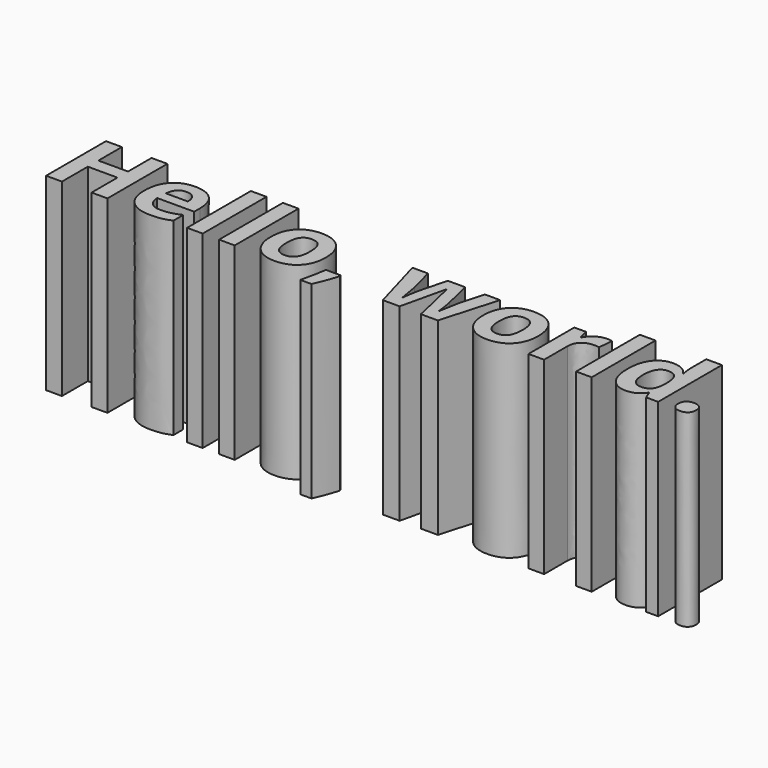
from build123d import *

# Parameters (mm, degrees)
F0_TEXT_SIZE = 27.7777777778
F1_DEPTH     = 50


# Not quite as in the source:
# - Text() gives the source's letters only with a copy of the font that has no kerning and outlines rounded to 1/6400 em; it was checked with that copy


with BuildPart() as f1:
    # F0 (on Top) → F1 (new body)
    with BuildSketch(Plane.XY):
        with Locations((-16.0339948229, -8.6685560189)):
            Text('Hello, world.', F0_TEXT_SIZE, font='Open Sans', font_style=FontStyle.BOLD, text_align=(TextAlign.LEFT, TextAlign.BOTTOM))
    extrude(amount=F1_DEPTH)


solid = f1.part
